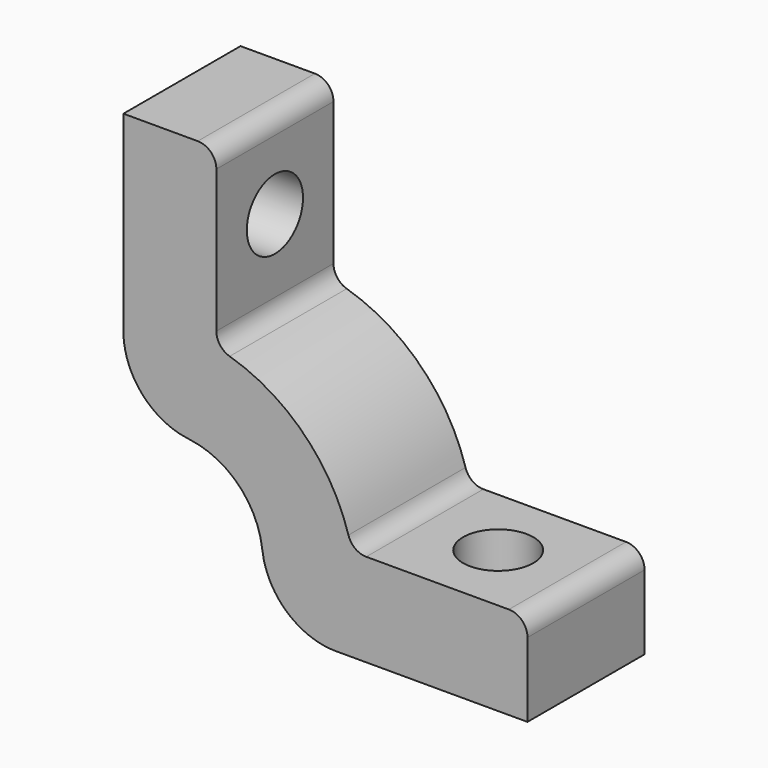
from build123d import *

# Parameters (mm, degrees)
F1_DEPTH = 10
F2_R     = 2.4
F3_DEPTH = 6.35
F7_R     = 5.08
F8_R     = 1.27


# Not quite as in the source:
# - a pattern or mirror of a feature is missing from the dataset's text; its kind, count and spacing are read off the source's solid


with BuildPart() as f1:
    # F0 (on Front) → F1 (new body)
    with BuildSketch(Plane.XZ):
        with BuildLine():
            ThreePointArc((0, 5.715), (4.0411152545, 4.0411152545), (5.715, 0))
            Line((5.715, 0), (5.715, -3.81))
            Line((5.715, -3.81), (23.7946015193, -3.81))
            Line((23.7946015193, -3.81), (23.7946015193, 2.54))
            Line((23.7946015193, 2.54), (11.7946015193, 2.54))
            ThreePointArc((11.7946015193, 2.54), (8.531243315, 8.531243315), (2.54, 11.7946015193))
            Line((2.54, 11.7946015193), (2.54, 23.7946015193))
            Line((2.54, 23.7946015193), (-3.81, 23.7946015193))
            Line((-3.81, 23.7946015193), (-3.81, 5.715))
            Line((-3.81, 5.715), (0, 5.715))
        make_face()
    extrude(amount=F1_DEPTH)

    # F2 (on face) → F3 (cut, through all)
    with BuildSketch(Plane.XY.offset(2.54)):
        with Locations((17.7946015193, -5)):
            Circle(F2_R)
    f3 = extrude(amount=-F3_DEPTH, mode=Mode.SUBTRACT)

    # F3_copies: F3 across plane
    add(f3.mirror(Plane(origin=(0, 0, 0), x_dir=(0.7071067812, 0, 0.7071067812), z_dir=(-0.7071067812, 0, 0.7071067812))), mode=Mode.SUBTRACT)

    # F7
    f7_edges = [f1.edges().sort_by_distance(p)[0] for p in [
        (-3.81, -5, 5.715),
        (5.715, -5, -3.81),
    ]]
    fillet(f7_edges, radius=F7_R)

    # F8
    f8_edges = [f1.edges().sort_by_distance(p)[0] for p in [
        (2.54, -5, 23.794602),
        (2.54, -5, 11.794602),
        (11.794602, -5, 2.54),
        (23.794602, -5, 2.54),
    ]]
    fillet(f8_edges, radius=F8_R)


solid = f1.part
